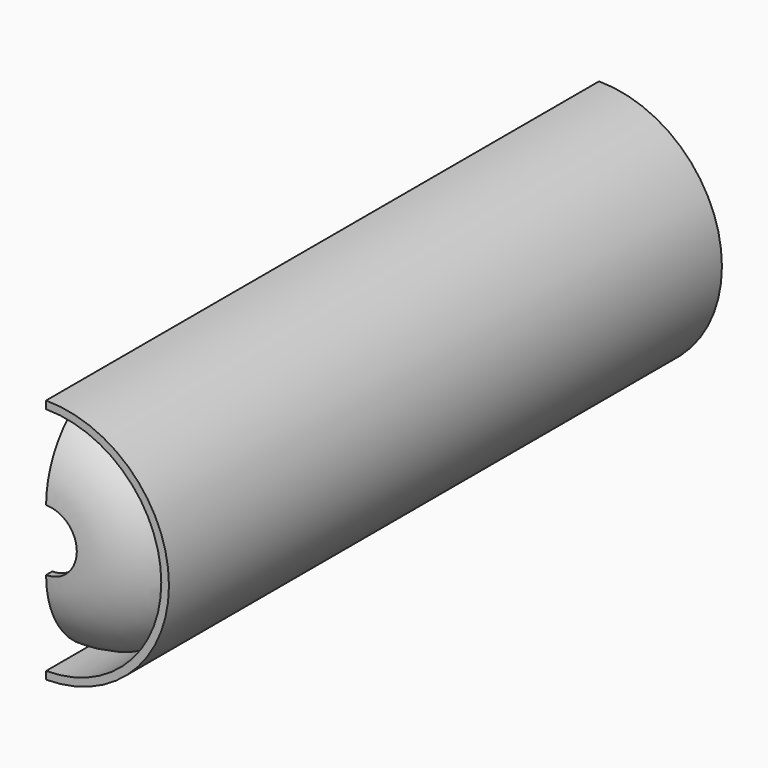
from build123d import *

# Parameters (mm, degrees)
F1_ANGLE = 180


# Not quite as in the source:
# - a feature names something its author has since deleted; it is built from what else it names


with BuildPart() as f1:
    # F0 (on Right) → F1 (revolve)
    with BuildSketch(Plane.YZ):
        with BuildLine():
            Line((86.8716222048, 33.384835436), (-3.1283777952, 33.384835436))
            Line((-3.1283777952, 33.384835436), (-3.1283777952, 32.384835436))
            Line((-3.1283777952, 32.384835436), (4.0757906815, 32.384835436))
            ThreePointArc((4.0757906815, 32.384835436), (-1.1670524657, 27.9594084914), (-3.1283777952, 21.384835436))
            Line((-3.1283777952, 21.384835436), (-2.1283777952, 21.384835436))
            ThreePointArc((-2.1283777952, 21.384835436), (1.0934476117, 29.1630100291), (8.8716222048, 32.384835436))
            Line((8.8716222048, 32.384835436), (71.8716222048, 32.384835436))
            ThreePointArc((71.8716222048, 32.384835436), (79.3046565784, 29.0966848666), (81.8716222048, 21.384835436))
            Line((81.8716222048, 21.384835436), (83.8716222048, 21.384835436))
            Line((83.8716222048, 21.384835436), (86.8716222048, 23.384835436))
            Line((86.8716222048, 23.384835436), (86.8716222048, 25.384835436))
            Line((86.8716222048, 25.384835436), (85.8716222048, 25.384835436))
            Line((85.8716222048, 25.384835436), (85.8716222048, 23.9200191945))
            Line((85.8716222048, 23.9200191945), (83.568846567, 22.384835436))
            Line((83.568846567, 22.384835436), (82.3074740727, 22.384835436))
            ThreePointArc((82.3074740727, 22.384835436), (80.8426391774, 28.2945551763), (76.3326351779, 32.384835436))
            Line((76.3326351779, 32.384835436), (86.8716222048, 32.384835436))
            Line((86.8716222048, 32.384835436), (86.8716222048, 33.384835436))
        make_face()
    revolve(axis=Axis((0, 40.3716222048, 17.384835436), (0, 1, 0)), revolution_arc=F1_ANGLE)


solid = f1.part
